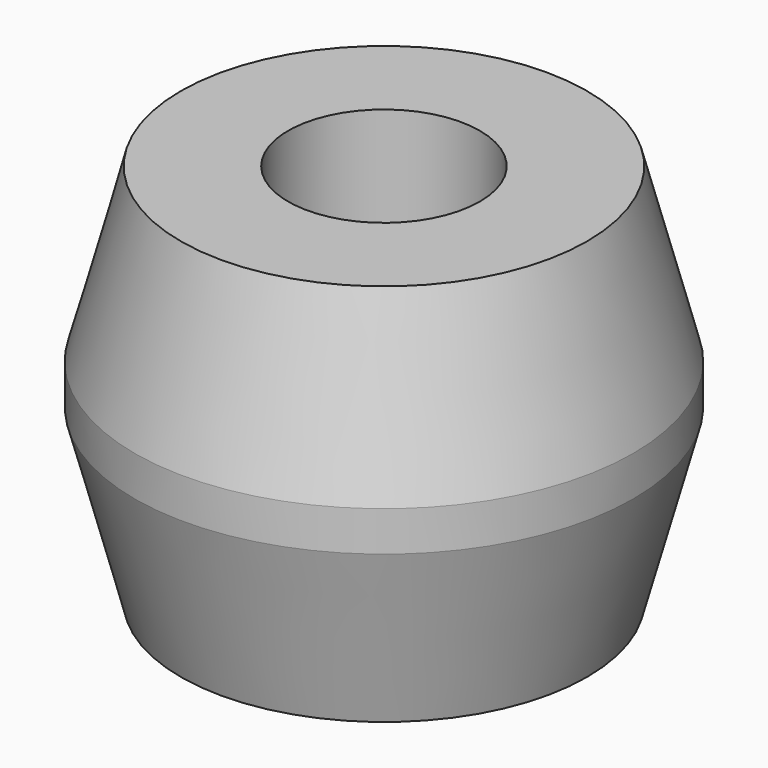
from build123d import *

# Parameters (mm, degrees)
F0_R       = 3.25
F0_R_2     = 2.9
F0_R_3     = 1.25
F1_DEPTH   = 5
F2_SIZE2   = 2.2392304845
F2_SIZE    = 0.6
F2_2_SIZE2 = 2.2392304845
F2_2_SIZE  = 0.6


with BuildPart() as f1:
    # F0 (on Top) → F1 (new body)
    with BuildSketch(Plane.XY):
        Circle(F0_R)
        Circle(F0_R_2, mode=Mode.SUBTRACT)
        Circle(F0_R_2)
        Circle(F0_R_3, mode=Mode.SUBTRACT)
    extrude(amount=F1_DEPTH)

    # F2
    f2_edges = [f1.edges().sort_by_distance(p)[0] for p in [
        (-3.25, 0, 5),
    ]]
    f2_side = f1.faces().sort_by_distance((-1.341924, 0, 5))[0]
    chamfer(f2_edges, length=F2_SIZE, length2=F2_SIZE2, reference=f2_side)

    # F2#2
    f2_2_edges = [f1.edges().sort_by_distance(p)[0] for p in [
        (-3.25, 0, 0),
    ]]
    f2_2_side = f1.faces().sort_by_distance((-1.341924, 0, 0))[0]
    chamfer(f2_2_edges, length=F2_2_SIZE, length2=F2_2_SIZE2, reference=f2_2_side)


solid = f1.part
